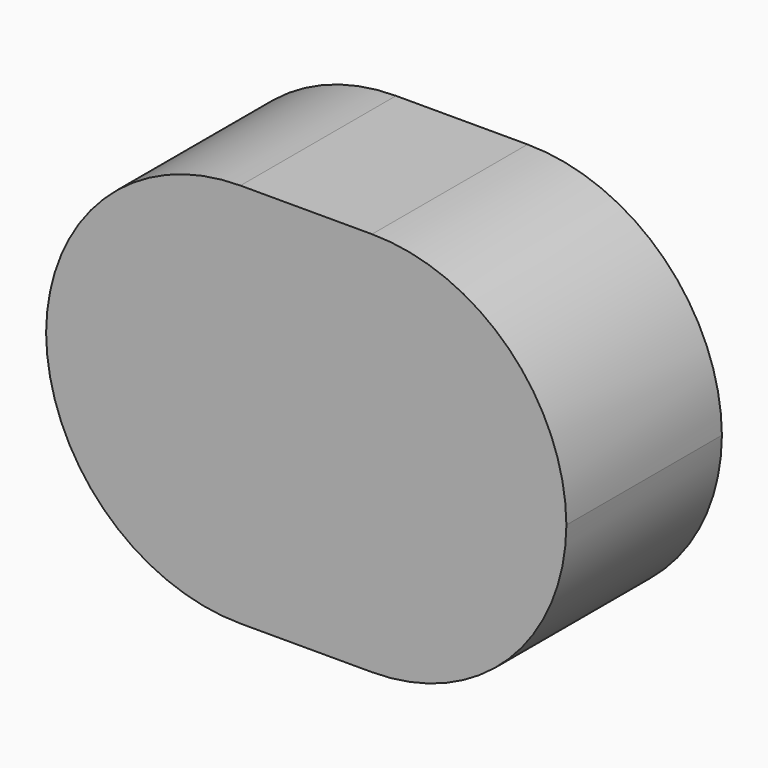
from build123d import *

# Parameters (mm, degrees)
F0_W        = 67.9875686765
F0_H        = 50.382964313
F1_DEPTH    = 25.4
F2_T1_DEPTH = 152.4


# Not quite as in the source:
# - a fillet or chamfer that OpenCascade refuses, or shapes differently, is made with other operations: its cross-section is extruded or revolved along the edge and cut away or added


with BuildPart() as f1:
    # F0 (on Front) → F1 (new body)
    with BuildSketch(Plane.XZ):
        with Locations((33.9937843382, 25.1914821565)):
            Rectangle(F0_W, F0_H)
    extrude(amount=F1_DEPTH)

    # F2: fillet of radius 25.4 on 4 edges, made by hand

    # F2_s2 → F2_t1 (cut)
    with BuildSketch(Plane.XZ.offset(-63.5)):
        with BuildLine():
            ThreePointArc((0, 24.982964313), (7.4394877579, 42.9434765552), (25.4, 50.382964313))
            Line((25.4, 50.382964313), (0, 50.382964313))
            Line((0, 50.382964313), (0, 24.982964313))
        make_face()
        with BuildLine():
            ThreePointArc((67.9875686765, 24.982964313), (60.5480809186, 42.9434765552), (42.5875686765, 50.382964313))
            Line((42.5875686765, 50.382964313), (67.9875686765, 50.382964313))
            Line((67.9875686765, 50.382964313), (67.9875686765, 24.982964313))
        make_face()
        with BuildLine():
            ThreePointArc((0, 25.4), (7.4394877579, 7.4394877579), (25.4, 0))
            Line((25.4, 0), (0, 0))
            Line((0, 0), (0, 25.4))
        make_face()
        with BuildLine():
            ThreePointArc((42.5875686765, 0), (60.5480809186, 7.4394877579), (67.9875686765, 25.4))
            Line((67.9875686765, 25.4), (67.9875686765, 0))
            Line((67.9875686765, 0), (42.5875686765, 0))
        make_face()
    extrude(amount=F2_T1_DEPTH, mode=Mode.SUBTRACT)


solid = f1.part
